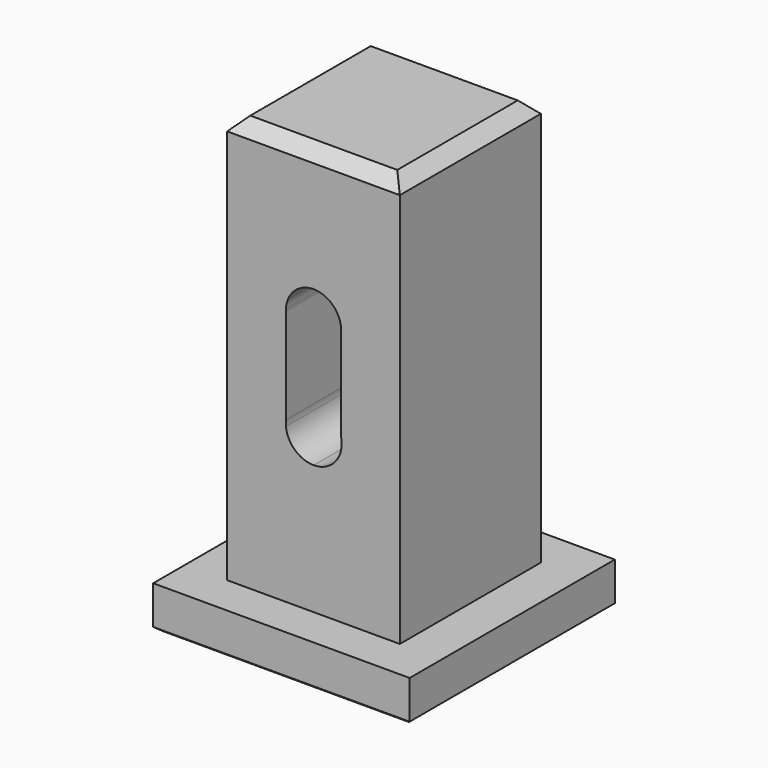
from build123d import *

# Parameters (mm, degrees)
F0_W        = 25.3882817924
F0_H        = 25.3883041441
F1_DEPTH    = 5.08
F2_W        = 17.0946475118
F2_H        = 17.4471139908
F3_DEPTH    = 45.466
F5_DEPTH    = 25.4
F6_DEPTH    = 25.4
F7_SIZE     = 1.27
F8_SIZE     = 1.27
F9_T1_DEPTH = 33.2988026177
F9_T3_DEPTH = 33.2988249694


# Not quite as in the source:
# - a fillet or chamfer that OpenCascade refuses, or shapes differently, is made with other operations: its cross-section is extruded or revolved along the edge and cut away or added


with BuildPart() as f1:
    # F0 (on Top) → F1 (new body)
    with BuildSketch(Plane.XY):
        Rectangle(F0_W, F0_H)
    extrude(amount=F1_DEPTH)

    # F2 (on Top) → F3 (join)
    with BuildSketch(Plane.XY):
        Rectangle(F2_W, F2_H)
    extrude(amount=F3_DEPTH)

    # F4 (on Front) → F5 (cut)
    with BuildSketch(Plane.XZ):
        with BuildLine():
            ThreePointArc((-2.7316187043, 20.3549675643), (-1.8326762864, 18.6002154817), (0.0056849059, 17.8876984864))
            Line((0.0056849059, 17.8876984864), (0.0386628839, 17.8876984864))
            ThreePointArc((0.0386628839, 17.8876984864), (1.7712415134, 18.5095830103), (2.7316187043, 20.0800112066))
            Line((2.7316187043, 20.0800112066), (2.7316187043, 21.236134693))
            Line((2.7316187043, 21.236134693), (2.7316187043, 30.2240438759))
            Line((2.7316187043, 30.2240438759), (2.7316187043, 30.752742663))
            ThreePointArc((2.7316187043, 30.752742663), (2.1863530417, 32.1452825707), (0.9908690064, 33.0437812954))
            Line((0.9908690064, 33.0437812954), (-0.9794991946, 33.0437812954))
            ThreePointArc((-0.9794991946, 33.0437812954), (-2.2272694516, 32.0741140874), (-2.7316187043, 30.5765103549))
            Line((-2.7316187043, 30.5765103549), (-2.7316187043, 30.4002761841))
            Line((-2.7316187043, 30.4002761841), (-2.7316187043, 20.9611783353))
            Line((-2.7316187043, 20.9611783353), (-2.7316187043, 20.3549675643))
        make_face()
        with BuildLine():
            ThreePointArc((-2.7316187043, 20.9611783353), (-2.7482496384, 20.6580729498), (-2.7316187043, 20.3549675643))
            Line((-2.7316187043, 20.3549675643), (-2.7316187043, 20.9611783353))
        make_face()
        with BuildLine():
            Line((2.7316187043, 21.236134693), (2.7316187043, 20.0800112066))
            ThreePointArc((2.7316187043, 20.0800112066), (2.7925974282, 20.6580729498), (2.7316187043, 21.236134693))
        make_face()
        with BuildLine():
            ThreePointArc((-2.7316187043, 30.5765103549), (-2.7330366343, 30.4883932695), (-2.7316187043, 30.4002761841))
            Line((-2.7316187043, 30.4002761841), (-2.7316187043, 30.5765103549))
        make_face()
        with BuildLine():
            Line((2.7316187043, 30.752742663), (2.7316187043, 30.2240438759))
            ThreePointArc((2.7316187043, 30.2240438759), (2.7444064461, 30.4883932695), (2.7316187043, 30.752742663))
        make_face()
        with BuildLine():
            ThreePointArc((0.9908690064, 33.0437812954), (0.0056849059, 33.2271148097), (-0.9794991946, 33.0437812954))
            Line((-0.9794991946, 33.0437812954), (0.9908690064, 33.0437812954))
        make_face()
    extrude(amount=-F5_DEPTH, mode=Mode.SUBTRACT)

    # F6 (cut): a face of the model
    f6_faces = [f1.faces().sort_by_distance(p)[0] for p in [
        (0.0051043388, 0, 25.5481593175),
    ]]
    extrude(f6_faces, amount=-F6_DEPTH, mode=Mode.SUBTRACT)

    # F7
    f7_edges = [f1.edges().sort_by_distance(p)[0] for p in [
        (0, -12.694152, 0),
        (12.694141, 0, 0),
        (-12.694141, 0, 0),
        (0, 12.694152, 0),
    ]]
    chamfer(f7_edges, length=F7_SIZE)

    # F8
    f8_edges = [f1.edges().sort_by_distance(p)[0] for p in [
        (0, 8.723557, 45.466),
        (-8.547324, 0, 45.466),
        (0, -8.723557, 45.466),
        (8.547324, 0, 45.466),
    ]]
    chamfer(f8_edges, length=F8_SIZE)

    # F9: fillet of radius 5.08 on 4 edges, made by hand

    # F9_s2 → F9_t1 (cut)
    with BuildSketch(Plane.YZ.offset(-16.6494013088)):
        with BuildLine():
            ThreePointArc((-12.6941520721, 1.27), (-11.1300991312, 0.3280951188), (-9.334047907, 0))
            Line((-9.334047907, 0), (-11.4241520721, 0))
            Line((-11.4241520721, 0), (-12.6941520721, 1.27))
        make_face()
        with BuildLine():
            ThreePointArc((12.6941520721, 1.27), (11.1300991312, 0.3280951188), (9.334047907, 0))
            Line((9.334047907, 0), (11.4241520721, 0))
            Line((11.4241520721, 0), (12.6941520721, 1.27))
        make_face()
    extrude(amount=F9_T1_DEPTH, mode=Mode.SUBTRACT)

    # F9_s4 → F9_t3 (cut)
    with BuildSketch(Plane.XZ.offset(-16.6494124847)):
        with BuildLine():
            ThreePointArc((12.6941408962, 1.27), (11.1300879554, 0.3280951188), (9.3340367311, 0))
            Line((9.3340367311, 0), (11.4241408962, 0))
            Line((11.4241408962, 0), (12.6941408962, 1.27))
        make_face()
        with BuildLine():
            ThreePointArc((-12.6941408962, 1.27), (-11.1300879554, 0.3280951188), (-9.3340367311, 0))
            Line((-9.3340367311, 0), (-11.4241408962, 0))
            Line((-11.4241408962, 0), (-12.6941408962, 1.27))
        make_face()
    extrude(amount=F9_T3_DEPTH, mode=Mode.SUBTRACT)


solid = f1.part
